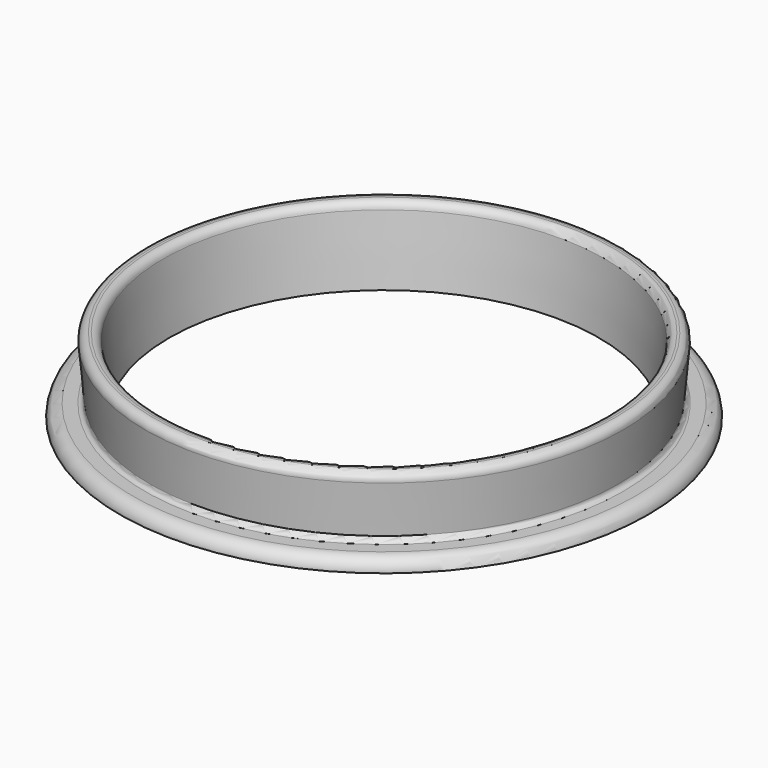
from build123d import *

# Parameters (mm, degrees)
F0_R      = 42
F0_R_2    = 36.5
F1_DEPTH  = 2
F4_R      = 42.35
F4_R_2    = 42
F5_DEPTH  = 2
F6_R      = 1.99999
F7_R      = 37.375
F7_R_2    = 34.5
F8_DEPTH  = 12
F8_TAPER  = -5
F9_R      = 38.4248639623
F10_DEPTH = 25
F11_R     = 34.5
F12_DEPTH = 25
F12_TAPER = -5
F13_R     = 1.25
F14_R     = 0.75


# Not quite as in the source:
# - a fillet or chamfer is up to 0.001 mm smaller than in the source, because OpenCascade refuses the exact size


with BuildPart() as f1:
    # F0 (on Top) → F1 (new body)
    with BuildSketch(Plane.XY):
        Circle(F0_R)
        Circle(F0_R_2, mode=Mode.SUBTRACT)
    extrude(amount=F1_DEPTH)

    # F2 (on Front) → F3 (revolve)
    with BuildSketch(Plane.XZ):
        with BuildLine():
            Line((36.5, 0), (36.5, 2))
            Line((36.5, 2), (35.5, 2))
            ThreePointArc((35.5, 2), (34.7928932188, 2.2928932188), (34.5, 3))
            Line((34.5, 3), (34.5, 14.1715728753))
            ThreePointArc((34.5, 14.1715728753), (34.6835034191, 14.7489231444), (35.1666666667, 15.1143819168))
            ThreePointArc((35.1666666667, 15.1143819168), (35.6547005384, 18.6329931619), (32.5, 17))
            Line((32.5, 17), (32.5, 2))
            ThreePointArc((32.5, 2), (33.0857864376, 0.5857864376), (34.5, 0))
            Line((34.5, 0), (36.5, 0))
        make_face()
    revolve(axis=Axis((0, 0, 63.5549128056), (0, 0, 1)))

    # F4 (on face) → F5 (join)
    with BuildSketch(Plane.XY.offset(2)):
        Circle(F4_R)
        Circle(F4_R_2, mode=Mode.SUBTRACT)
    extrude(amount=-F5_DEPTH)

    # F6 (radius 2 in the source; OpenCascade refuses exactly that, so slightly less here)
    f6_edges = [f1.edges().sort_by_distance(p)[0] for p in [
        (-42.35, 0, 2),
    ]]
    fillet(f6_edges, radius=F6_R)

    # F7 (on face) → F8 (join)
    with BuildSketch(Plane(origin=(0, 0, 0), x_dir=(1, 0, 0), z_dir=(0, 0, -1))):
        Circle(F7_R)
        Circle(F7_R_2, mode=Mode.SUBTRACT)
    extrude(amount=-F8_DEPTH, taper=F8_TAPER)

    # F9 (on face) → F10 (cut)
    with BuildSketch(Plane.XY.offset(12)):
        Circle(F9_R)
    extrude(amount=F10_DEPTH, mode=Mode.SUBTRACT)

    # F11 (on face) → F12 (cut)
    with BuildSketch(Plane(origin=(0, 0, 0), x_dir=(1, 0, 0), z_dir=(0, 0, -1))):
        Circle(F11_R)
    extrude(amount=-F12_DEPTH, taper=F12_TAPER, mode=Mode.SUBTRACT)

    # F13
    f13_edges = [f1.edges().sort_by_distance(p)[0] for p in [
        (-38.424864, 0, 12),
        (-35.549864, 0, 12),
    ]]
    fillet(f13_edges, radius=F13_R)

    # F14
    f14_edges = [f1.edges().sort_by_distance(p)[0] for p in [
        (-37.549977, 0, 2),
    ]]
    fillet(f14_edges, radius=F14_R)


solid = f1.part
